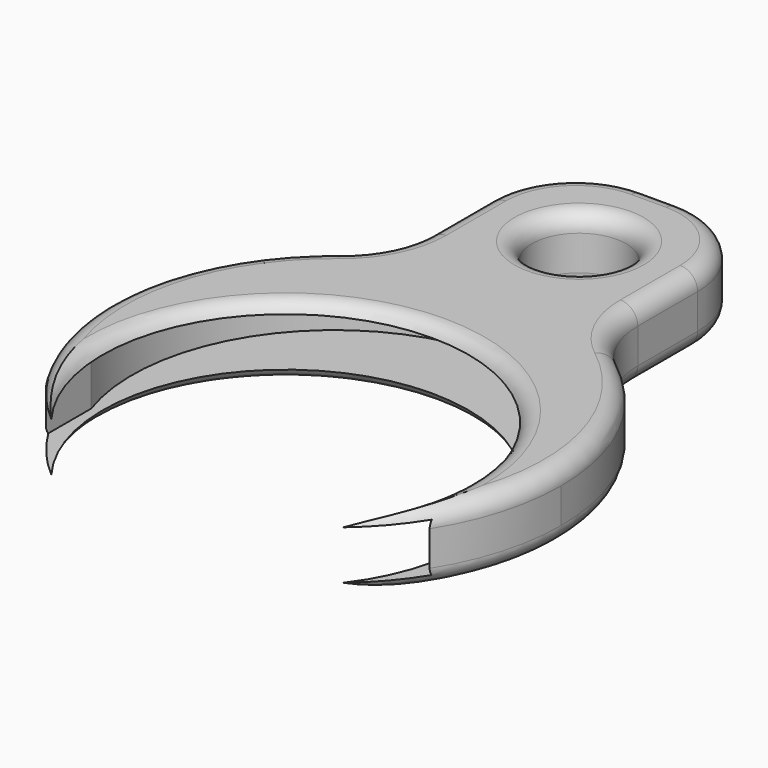
from build123d import *

# Parameters (mm, degrees)
F0_R         = 2.7
F1_DEPTH     = 2
F2_R         = 5
F3_R         = 1
F4_R         = 10.5
F5_DEPTH     = 4.001
F7_DEPTH     = 1.4
F8_T1_DEPTH  = 4.2847557459
F8_T3_DEPTH  = 2
F8_T6_ANGLE  = 114.6351015634
F8_T8_ANGLE  = 52.3301130357
F8_T10_ANGLE = 90
F8_T12_ANGLE = 114.6351015634
F8_T14_ANGLE = 283.5812269482
F8_T16_ANGLE = 283.5812269482
F8_T18_ANGLE = 52.3301130357
F8_T20_ANGLE = 90
F8_T22_ANGLE = 90
F8_T24_ANGLE = 52.3301130357
F8_T26_ANGLE = 114.6351015634
F8_T28_ANGLE = 90
F8_T30_ANGLE = 52.3301130357
F8_T32_ANGLE = 114.6351015634


# Not quite as in the source:
# - a fillet or chamfer that OpenCascade refuses, or shapes differently, is made with other operations: its cross-section is extruded or revolved along the edge and cut away or added


with BuildPart() as f1:
    # F0 (on Top) → F1 (new body, symmetric)
    with BuildSketch(Plane.XY):
        with BuildLine():
            ThreePointArc((-6, 11.5325625947), (-6.7453687816, -11.1130553854), (13, 0))
            ThreePointArc((13, 0), (11.1130553854, 6.7453687816), (6, 11.5325625947))
            Line((6, 11.5325625947), (-6, 11.5325625947))
        make_face()
        with BuildLine():
            Line((-6, 11.5325625947), (6, 11.5325625947))
            ThreePointArc((6, 11.5325625947), (0, 13), (-6, 11.5325625947))
        make_face()
        with BuildLine():
            ThreePointArc((-6, 11.5325625947), (0, 13), (6, 11.5325625947))
            Line((6, 11.5325625947), (6, 23.5325625947))
            Line((6, 23.5325625947), (-6, 23.5325625947))
            Line((-6, 23.5325625947), (-6, 11.5325625947))
        make_face()
        with Locations((0, 17.5325625947)):
            Circle(F0_R, mode=Mode.SUBTRACT)
    extrude(amount=F1_DEPTH, both=True)

    # F2
    f2_edges = [f1.edges().sort_by_distance(p)[0] for p in [
        (6, 11.532563, 0),
        (6, 23.532563, 0),
        (-6, 23.532563, 0),
        (-6, 11.532563, 0),
    ]]
    fillet(f2_edges, radius=F2_R)

    # F3
    f3_edges = [f1.edges().sort_by_distance(p)[0] for p in [
        (-2.7, 17.532563, -2),
        (-2.7, 17.532563, 2),
    ]]
    fillet(f3_edges, radius=F3_R)

    # F4 (on face) → F5 (cut, through all)
    with BuildSketch(Plane(origin=(0, 0, -2), x_dir=(1, 0, 0), z_dir=(0, 0, -1))):
        with Locations((0, 3.5)):
            Circle(F4_R)
    extrude(amount=-F5_DEPTH, mode=Mode.SUBTRACT)

    # F6 (on Top) → F7 (cut, symmetric)
    with BuildSketch(Plane.XY):
        with BuildLine():
            ThreePointArc((11, -3.6981110043), (11.452751307, -1.8736361707), (11.605, 0))
            ThreePointArc((11.605, 0), (-1.8736361707, 11.452751307), (-11, -3.6981110043))
            Line((-11, -3.6981110043), (11, -3.6981110043))
        make_face()
        with BuildLine():
            Line((11, -3.6981110043), (-11, -3.6981110043))
            ThreePointArc((-11, -3.6981110043), (0, -11.605), (11, -3.6981110043))
        make_face()
        with BuildLine():
            ThreePointArc((11, -3.6981110043), (0, -11.605), (-11, -3.6981110043))
            Line((-11, -3.6981110043), (-11, -14.5566218919))
            Line((-11, -14.5566218919), (11, -14.5566218919))
            Line((11, -14.5566218919), (11, -3.6981110043))
        make_face()
    extrude(amount=F7_DEPTH, both=True, mode=Mode.SUBTRACT)

    # F8: fillet of radius 1 on 20 edges, made by hand

    # F8_s2 → F8_t1 (cut)
    with BuildSketch(Plane.XZ.offset(-18.5325625947)):
        with BuildLine():
            ThreePointArc((6, 1), (5.7071067812, 1.7071067812), (5, 2))
            Line((5, 2), (6, 2))
            Line((6, 2), (6, 1))
        make_face()
        with BuildLine():
            ThreePointArc((5, -2), (5.7071067812, -1.7071067812), (6, -1))
            Line((6, -1), (6, -2))
            Line((6, -2), (5, -2))
        make_face()
        with BuildLine():
            ThreePointArc((-5, -2), (-5.7071067812, -1.7071067812), (-6, -1))
            Line((-6, -1), (-6, -2))
            Line((-6, -2), (-5, -2))
        make_face()
        with BuildLine():
            ThreePointArc((-6, 1), (-5.7071067812, 1.7071067812), (-5, 2))
            Line((-5, 2), (-6, 2))
            Line((-6, 2), (-6, 1))
        make_face()
    extrude(amount=F8_T1_DEPTH, mode=Mode.SUBTRACT)

    # F8_s4 → F8_t3 (cut)
    with BuildSketch(Plane.YZ.offset(-1)):
        with BuildLine():
            ThreePointArc((22.5325625947, -2), (23.2396693759, -1.7071067812), (23.5325625947, -1))
            Line((23.5325625947, -1), (23.5325625947, -2))
            Line((23.5325625947, -2), (22.5325625947, -2))
        make_face()
        with BuildLine():
            ThreePointArc((23.5325625947, 1), (23.2396693759, 1.7071067812), (22.5325625947, 2))
            Line((22.5325625947, 2), (23.5325625947, 2))
            Line((23.5325625947, 2), (23.5325625947, 1))
        make_face()
    extrude(amount=F8_T3_DEPTH, mode=Mode.SUBTRACT)

    # F8_s5 → F8_t6 (revolve, cut)
    with BuildSketch(Plane(origin=(0, 0, 0), x_dir=(0, 0, 1), z_dir=(-0.8854340944, -0.4647649561, 0))):
        with BuildLine():
            ThreePointArc((1, -13), (1.7071067812, -12.7071067812), (2, -12))
            Line((2, -12), (2, -13))
            Line((2, -13), (1, -13))
        make_face()
    revolve(axis=Axis((0, 0, 2), (0, 0, 1)), revolution_arc=F8_T6_ANGLE, mode=Mode.SUBTRACT)

    # F8_s7 → F8_t8 (revolve, cut)
    with BuildSketch(Plane.XZ.offset(-14.2478068488)):
        with BuildLine():
            ThreePointArc((6, 1), (5.7071067812, 1.7071067812), (5, 2))
            Line((5, 2), (6, 2))
            Line((6, 2), (6, 1))
        make_face()
    revolve(axis=Axis((11, 14.2478068488, 2), (0, 0, 1)), revolution_arc=F8_T8_ANGLE, mode=Mode.SUBTRACT)

    # F8_s9 → F8_t10 (revolve, cut)
    with BuildSketch(Plane.XZ.offset(-18.5325625947)):
        with BuildLine():
            ThreePointArc((6, 1), (5.7071067812, 1.7071067812), (5, 2))
            Line((5, 2), (6, 2))
            Line((6, 2), (6, 1))
        make_face()
    revolve(axis=Axis((1, 18.5325625947, 2), (0, 0, 1)), revolution_arc=F8_T10_ANGLE, mode=Mode.SUBTRACT)

    # F8_s11 → F8_t12 (revolve, cut)
    with BuildSketch(Plane(origin=(0, 0, 0), x_dir=(0, 0, 1), z_dir=(0.7915448249, 0.6111111111, 0))):
        with BuildLine():
            ThreePointArc((-2, -12), (-1.7071067812, -12.7071067812), (-1, -13))
            Line((-1, -13), (-2, -13))
            Line((-2, -13), (-2, -12))
        make_face()
    revolve(axis=Axis((0, 0, -2), (0, 0, 1)), revolution_arc=F8_T12_ANGLE, mode=Mode.SUBTRACT)

    # F8_s13 → F8_t14 (revolve, cut)
    with BuildSketch(Plane(origin=(-1.7010664879, -1.3390586371, 0), x_dir=(0, 0, 1), z_dir=(-0.7857555714, -0.6185371307, 0))):
        with BuildLine():
            ThreePointArc((-2, -14.1666596389), (-1.8366600265, -13.6189370814), (-1.4, -13.2501444999))
            Line((-1.4, -13.2501444999), (-2, -13.2501444999))
            Line((-2, -13.2501444999), (-2, -14.1666596389))
        make_face()
    revolve(axis=Axis((0, -3.5, -2), (0, 0, 1)), revolution_arc=F8_T14_ANGLE, mode=Mode.SUBTRACT)

    # F8_s15 → F8_t16 (revolve, cut)
    with BuildSketch(Plane(origin=(-1.7010664879, -1.3390586371, 0), x_dir=(0, 0, 1), z_dir=(-0.7857555714, -0.6185371307, 0))):
        with BuildLine():
            ThreePointArc((2, -14.1666596389), (1.8366600265, -13.6189370814), (1.4, -13.2501444999))
            Line((1.4, -13.2501444999), (2, -13.2501444999))
            Line((2, -13.2501444999), (2, -14.1666596389))
        make_face()
    revolve(axis=Axis((0, -3.5, 2), (0, 0, 1)), revolution_arc=F8_T16_ANGLE, mode=Mode.SUBTRACT)

    # F8_s17 → F8_t18 (revolve, cut)
    with BuildSketch(Plane.XZ.offset(-14.2478068488)):
        with BuildLine():
            ThreePointArc((5, -2), (5.7071067812, -1.7071067812), (6, -1))
            Line((6, -1), (6, -2))
            Line((6, -2), (5, -2))
        make_face()
    revolve(axis=Axis((11, 14.2478068488, -2), (0, 0, 1)), revolution_arc=F8_T18_ANGLE, mode=Mode.SUBTRACT)

    # F8_s19 → F8_t20 (revolve, cut)
    with BuildSketch(Plane.XZ.offset(-18.5325625947)):
        with BuildLine():
            ThreePointArc((5, -2), (5.7071067812, -1.7071067812), (6, -1))
            Line((6, -1), (6, -2))
            Line((6, -2), (5, -2))
        make_face()
    revolve(axis=Axis((1, 18.5325625947, -2), (0, 0, 1)), revolution_arc=F8_T20_ANGLE, mode=Mode.SUBTRACT)

    # F8_s21 → F8_t22 (revolve, cut)
    with BuildSketch(Plane.XZ.offset(-18.5325625947)):
        with BuildLine():
            ThreePointArc((-5, -2), (-5.7071067812, -1.7071067812), (-6, -1))
            Line((-6, -1), (-6, -2))
            Line((-6, -2), (-5, -2))
        make_face()
    revolve(axis=Axis((-1, 18.5325625947, -2), (0, 0, -1)), revolution_arc=F8_T22_ANGLE, mode=Mode.SUBTRACT)

    # F8_s23 → F8_t24 (revolve, cut)
    with BuildSketch(Plane(origin=(0, 0, 0), x_dir=(0, 0, 1), z_dir=(-0.7915448249, -0.6111111111, 0))):
        with BuildLine():
            ThreePointArc((-2, 12), (-1.7071067812, 12.7071067812), (-1, 13))
            Line((-1, 13), (-2, 13))
            Line((-2, 13), (-2, 12))
        make_face()
    revolve(axis=Axis((-11, 14.2478068488, -2), (0, 0, 1)), revolution_arc=F8_T24_ANGLE, mode=Mode.SUBTRACT)

    # F8_s25 → F8_t26 (revolve, cut)
    with BuildSketch(Plane(origin=(0, 0, 0), x_dir=(0, 0, 1), z_dir=(-0.8854340944, -0.4647649561, 0))):
        with BuildLine():
            ThreePointArc((-2, -12), (-1.7071067812, -12.7071067812), (-1, -13))
            Line((-1, -13), (-2, -13))
            Line((-2, -13), (-2, -12))
        make_face()
    revolve(axis=Axis((0, 0, -2), (0, 0, 1)), revolution_arc=F8_T26_ANGLE, mode=Mode.SUBTRACT)

    # F8_s27 → F8_t28 (revolve, cut)
    with BuildSketch(Plane.XZ.offset(-18.5325625947)):
        with BuildLine():
            ThreePointArc((-6, 1), (-5.7071067812, 1.7071067812), (-5, 2))
            Line((-5, 2), (-6, 2))
            Line((-6, 2), (-6, 1))
        make_face()
    revolve(axis=Axis((-1, 18.5325625947, 2), (0, 0, -1)), revolution_arc=F8_T28_ANGLE, mode=Mode.SUBTRACT)

    # F8_s29 → F8_t30 (revolve, cut)
    with BuildSketch(Plane(origin=(0, 0, 0), x_dir=(0, 0, 1), z_dir=(-0.7915448249, -0.6111111111, 0))):
        with BuildLine():
            ThreePointArc((1, 13), (1.7071067812, 12.7071067812), (2, 12))
            Line((2, 12), (2, 13))
            Line((2, 13), (1, 13))
        make_face()
    revolve(axis=Axis((-11, 14.2478068488, 2), (0, 0, 1)), revolution_arc=F8_T30_ANGLE, mode=Mode.SUBTRACT)

    # F8_s31 → F8_t32 (revolve, cut)
    with BuildSketch(Plane(origin=(0, 0, 0), x_dir=(0, 0, 1), z_dir=(0.7915448249, 0.6111111111, 0))):
        with BuildLine():
            ThreePointArc((1, -13), (1.7071067812, -12.7071067812), (2, -12))
            Line((2, -12), (2, -13))
            Line((2, -13), (1, -13))
        make_face()
    revolve(axis=Axis((0, 0, 2), (0, 0, 1)), revolution_arc=F8_T32_ANGLE, mode=Mode.SUBTRACT)


solid = f1.part
